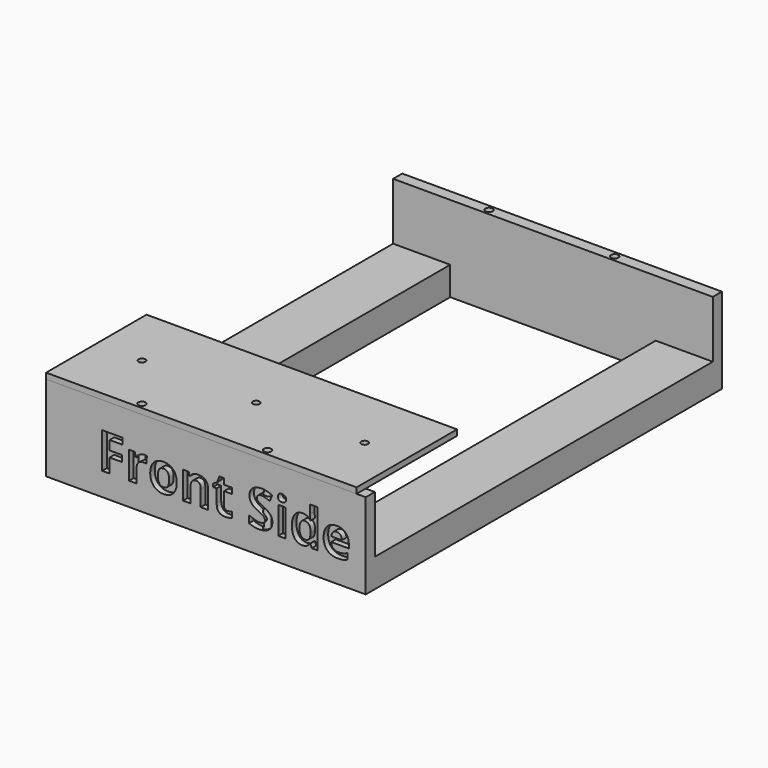
from build123d import *

# Parameters (mm, degrees)
F0_W         = 8
F0_H         = 10
F0_R         = 3.25
F1_DEPTH     = 75
F0_W_2       = 50
F0_H_2       = 270
F0_H_3       = 100
F0_R_2       = 3
F0_W_3       = 42
F2_DEPTH     = 25
F3_TEXT_SIZE = 43.9100691842
F4_DEPTH     = 5
F5_START     = 75
F0_W_4       = 180
F5_DEPTH     = 5


# Not quite as in the source:
# - Text() gives the source's letters only with a copy of the font that has no kerning and outlines rounded to 1/6400 em; it was checked with that copy


with BuildPart() as f1:
    # F0 (on Top) → F1 (new body)
    with BuildSketch(Plane.XY):
        with Locations((-4, 5)):
            Rectangle(F0_W, F0_H)
        Polygon((-280, 0), (-8, 0), (-8, 10), (-50, 10), (-230, 10), (-280, 10), align=None)
        with Locations((-200, 5)):
            Circle(F0_R, mode=Mode.SUBTRACT)
        with Locations((-90, 5)):
            Circle(F0_R, mode=Mode.SUBTRACT)
    extrude(amount=F1_DEPTH)



with BuildPart() as f1b:
    # F0 (on Top) → F1, piece 2 (new body)
    with BuildSketch(Plane.XY):
        Polygon((-50, 380), (0, 380), (0, 390), (-280, 390), (-280, 380), (-230, 380), align=None)
        with Locations((-200, 385)):
            Circle(F0_R, mode=Mode.SUBTRACT)
        with Locations((-90, 385)):
            Circle(F0_R, mode=Mode.SUBTRACT)
    extrude(amount=F1_DEPTH)


with BuildPart() as f1_1:
    add(f1.part)

    add(f1b.part)  # F2 merges F1b
    # F0 (on Top) → F2 (join)
    with BuildSketch(Plane.XY):
        with Locations((-255, 245)):
            Rectangle(F0_W_2, F0_H_2)
        with Locations((-255, 60)):
            Rectangle(F0_W_2, F0_H_3)
        with Locations((-240, 55)):
            Circle(F0_R_2, mode=Mode.SUBTRACT)
        Polygon((-8, 10), (0, 10), (0, 380), (-50, 380), (-50, 110), (-8, 110), align=None)
        with Locations((-29, 60)):
            Rectangle(F0_W_3, F0_H_3)
        with Locations((-45, 55)):
            Circle(F0_R_2, mode=Mode.SUBTRACT)
        with Locations((-240, 55)):
            Circle(F0_R_2)
        with Locations((-45, 55)):
            Circle(F0_R_2)
    extrude(amount=F2_DEPTH)

    # F3 (on face) → F4 (cut)
    with BuildSketch(Plane.XZ):
        with Locations((-234.7982516512, 20.2794857323)):
            Text('Front Side', F3_TEXT_SIZE, font='Open Sans', font_style=FontStyle.BOLD, text_align=(TextAlign.LEFT, TextAlign.BOTTOM))
    extrude(amount=-F4_DEPTH, mode=Mode.SUBTRACT)


with BuildPart() as f5:
    # F0 (on Top) → F5 (new body)
    with BuildSketch(Plane.XY.offset(F5_START)):
        with Locations((-255, 60)):
            Rectangle(F0_W_2, F0_H_3)
        with Locations((-240, 55)):
            Circle(F0_R_2, mode=Mode.SUBTRACT)
        with Locations((-140, 60)):
            Rectangle(F0_W_4, F0_H_3)
        with Locations((-140, 55)):
            Circle(F0_R_2, mode=Mode.SUBTRACT)
        with Locations((-29, 60)):
            Rectangle(F0_W_3, F0_H_3)
        with Locations((-45, 55)):
            Circle(F0_R_2, mode=Mode.SUBTRACT)
        Polygon((-280, 0), (-8, 0), (-8, 10), (-50, 10), (-230, 10), (-280, 10), align=None)
        with Locations((-200, 5)):
            Circle(F0_R, mode=Mode.SUBTRACT)
        with Locations((-90, 5)):
            Circle(F0_R, mode=Mode.SUBTRACT)
    extrude(amount=F5_DEPTH)


solid = Compound([f1_1.part, f5.part])
